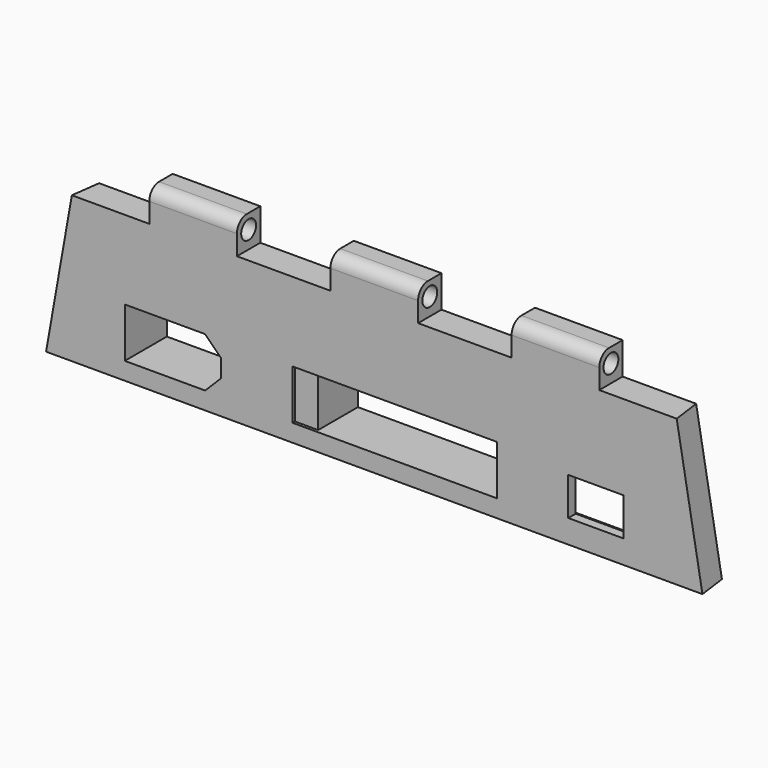
from build123d import *

# Parameters (mm, degrees)
F0_W       = 31
F0_H       = 8.5
F0_W_2     = 9.5
F0_H_2     = 6.5
F1_DEPTH   = 5
F2_W       = 4
F2_H       = 8.5
F3_DEPTH   = 0.5
F5_DEPTH   = 3.4125
F7_SIZE2   = 0.658252
F7_SIZE    = 4.99999
F7_2_SIZE2 = 0.658252
F7_2_SIZE  = 4.99999
F8_W       = 35
F8_H       = 12.5
F8_W_2     = 31
F8_H_2     = 8.5
F9_DEPTH   = 4
F11_DEPTH  = 4
F12_W      = 15
F12_H      = 5
F13_DEPTH  = 5.5
F14_R      = 1.5875
F15_DEPTH  = 94.6591745177
F16_R      = 2.1


# Not quite as in the source:
# - a fillet or chamfer is up to 0.001 mm smaller than in the source, because OpenCascade refuses the exact size
# - a length typed as a fraction of an inch, garbled in the dataset ("3 / 203.2 mm" for 3/8 in), is restored


with BuildPart() as f1:
    # F0 (on Front) → F1 (new body)
    with BuildSketch(Plane.XZ):
        Polygon((46.25, 17.75), (-57.25, 17.75), (-61.6581745177, -7.25), (50.6581745177, -7.25), align=None)
        Polygon((-48.1899019538, 4.25), (-34.4399019538, 4.25), (-31.6899019538, 1.5), (-31.6899019538, -1.5), (-34.4399019538, -4.25), (-48.1899019538, -4.25), align=None, mode=Mode.SUBTRACT)
        Rectangle(F0_W, F0_H, mode=Mode.SUBTRACT)
        with Locations((32.4399019538, 0)):
            Rectangle(F0_W_2, F0_H_2, mode=Mode.SUBTRACT)
    extrude(amount=-F1_DEPTH)

    # F2 (on face) → F3 (cut)
    with BuildSketch(Plane.XZ):
        with Locations((-17.5, 0)):
            Rectangle(F2_W, F2_H)
    extrude(amount=-F3_DEPTH, mode=Mode.SUBTRACT)

    # F4 (on face) → F5 (cut)
    with BuildSketch(Plane(origin=(0, 5, 0), x_dir=(-1, 0, 0), z_dir=(0, 1, 0))):
        Polygon((-22.1211519538, -5.3578125), (-22.1211519538, 5.3578125), (-42.7586519538, 5.3578125), (-42.7586519538, -5.3578125), align=None)
    extrude(amount=-F5_DEPTH, mode=Mode.SUBTRACT)

    # F7 (size 5 and 0.6582624879 in the source; OpenCascade refuses exactly that, so slightly less here)
    f7_edges = [f1.edges().sort_by_distance(p)[0] for p in [
        (-59.454087, 5, 5.25),
    ]]
    f7_side = f1.faces().sort_by_distance((-59.454087, 2.5, 5.25))[0]
    chamfer(f7_edges, length=F7_SIZE, length2=F7_SIZE2, reference=f7_side)

    # F7#2 (size 5 and 0.6582624879 in the source; OpenCascade refuses exactly that, so slightly less here)
    f7_2_edges = [f1.edges().sort_by_distance(p)[0] for p in [
        (48.454087, 5, 5.25),
    ]]
    f7_2_side = f1.faces().sort_by_distance((48.454087, 2.5, 5.25))[0]
    chamfer(f7_2_edges, length=F7_2_SIZE, length2=F7_2_SIZE2, reference=f7_2_side)

    # F8 (on face) → F9 (join)
    with BuildSketch(Plane(origin=(0, 5, 0), x_dir=(-1, 0, 0), z_dir=(0, 1, 0))):
        Rectangle(F8_W, F8_H)
        Rectangle(F8_W_2, F8_H_2, mode=Mode.SUBTRACT)
    extrude(amount=F9_DEPTH)

    # F10 (on face) → F11 (join)
    with BuildSketch(Plane(origin=(0, 5, 0), x_dir=(-1, 0, 0), z_dir=(0, 1, 0))):
        Polygon((50.1899019538, 6.25), (33.611474829, 6.25), (29.6899019538, 2.3284271247), (29.6899019538, -2.3284271247), (33.611474829, -6.25), (50.1899019538, -6.25), align=None)
        Polygon((31.6899019538, 1.5), (34.4399019538, 4.25), (48.1899019538, 4.25), (48.1899019538, -4.25), (34.4399019538, -4.25), (31.6899019538, -1.5), align=None, mode=Mode.SUBTRACT)
    extrude(amount=F11_DEPTH)

    # F12 (on face) → F13 (join)
    with BuildSketch(Plane.XY.offset(17.75)):
        with Locations((-36.5, 2.5)):
            Rectangle(F12_W, F12_H)
        with Locations((25.5, 2.5)):
            Rectangle(F12_W, F12_H)
        with Locations((-5.5, 2.5)):
            Rectangle(F12_W, F12_H)
    extrude(amount=F13_DEPTH)

    # F14 (on face) → F15 (cut, through all)
    with BuildSketch(Plane.YZ.offset(33)):
        with Locations((2.5, 20.75)):
            Circle(F14_R)
    extrude(amount=-F15_DEPTH, mode=Mode.SUBTRACT)

    # F16
    f16_edges = [f1.edges().sort_by_distance(p)[0] for p in [
        (-36.5, 0, 23.25),
        (-5.5, 0, 23.25),
        (25.5, 0, 23.25),
    ]]
    fillet(f16_edges, radius=F16_R)


solid = f1.part
